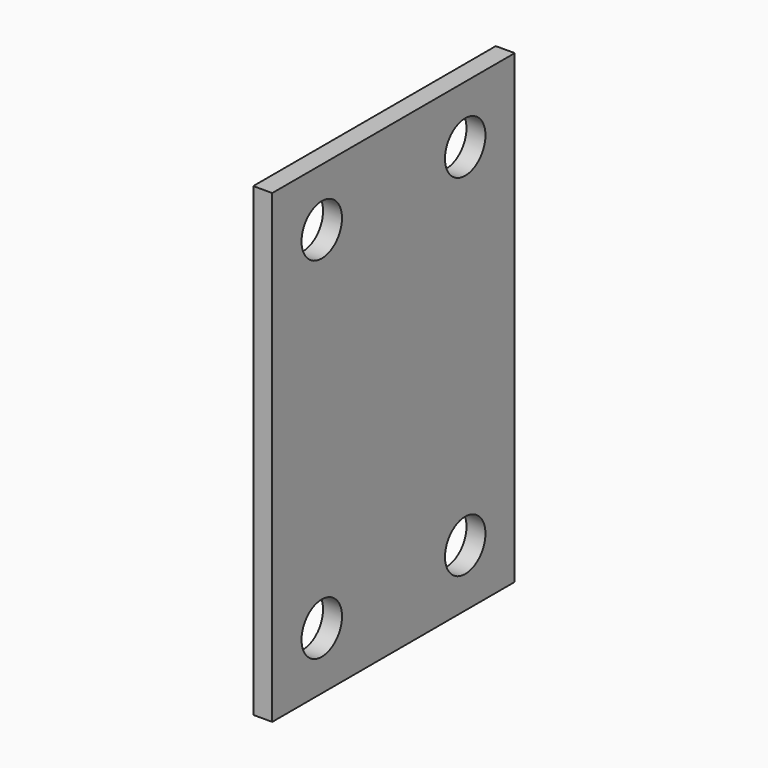
from build123d import *

# Parameters (mm, degrees)
F0_W     = 76.073
F0_H     = 116.84
F0_R     = 6.35
F1_DEPTH = 4.7625


# Not quite as in the source:
# - a length typed as a fraction of an inch, garbled in the dataset ("3 / 203.2 mm" for 3/8 in), is restored


with BuildPart() as f1:
    # F0 (on Right) → F1 (new body)
    with BuildSketch(Plane.YZ):
        Rectangle(F0_W, F0_H)
        with Locations((-22.5, -44)):
            Circle(F0_R, mode=Mode.SUBTRACT)
        with Locations((22.5, -44)):
            Circle(F0_R, mode=Mode.SUBTRACT)
        with Locations((-22.5, 44)):
            Circle(F0_R, mode=Mode.SUBTRACT)
        with Locations((22.5, 44)):
            Circle(F0_R, mode=Mode.SUBTRACT)
    extrude(amount=F1_DEPTH)


solid = f1.part
